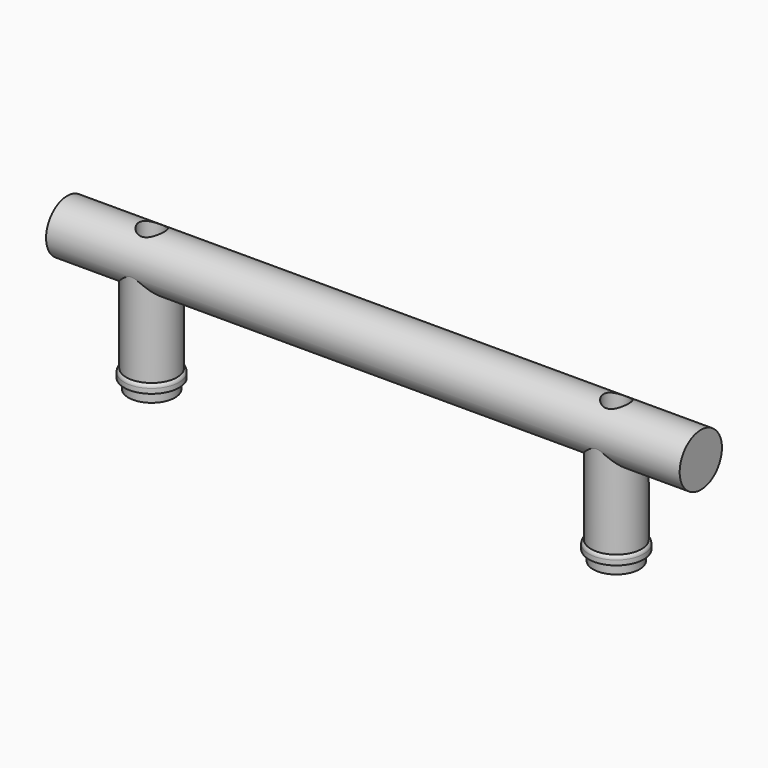
from build123d import *

# Parameters (mm, degrees)
F0_R     = 6
F0_R_2   = 5.5
F0_R_3   = 3
F1_DEPTH = 25
F0_R_4   = 6.5
F2_DEPTH = 2
F0_R_5   = 1.5
F3_DEPTH = 2.4
F4_R     = 6.25
F5_DEPTH = 75
F6_DEPTH = 40


# Not quite as in the source:
# - a fillet or chamfer that OpenCascade refuses, or shapes differently, is made with other operations: its cross-section is extruded or revolved along the edge and cut away or added


with BuildPart() as f1:
    # F0 (on Top) → F1 (new body)
    with BuildSketch(Plane.XY):
        with Locations((-55, 0)):
            Circle(F0_R)
        with Locations((-55, 0)):
            Circle(F0_R_2, mode=Mode.SUBTRACT)
        with Locations((-55, 0)):
            Circle(F0_R_2)
        with Locations((-55, 0)):
            Circle(F0_R_3, mode=Mode.SUBTRACT)
    extrude(amount=F1_DEPTH)

    # F0 (on Top) → F2 (join)
    with BuildSketch(Plane.XY):
        with Locations((-55, 0)):
            Circle(F0_R_4)
        with Locations((-55, 0)):
            Circle(F0_R, mode=Mode.SUBTRACT)
    extrude(amount=F2_DEPTH)

    # F0 (on Top) → F3 (join)
    with BuildSketch(Plane.XY):
        with Locations((-55, 0)):
            Circle(F0_R_2)
        with Locations((-55, 0)):
            Circle(F0_R_3, mode=Mode.SUBTRACT)
        with Locations((-55, 0)):
            Circle(F0_R_3)
        with Locations((-55, 0)):
            Circle(F0_R_5, mode=Mode.SUBTRACT)
    extrude(amount=-F3_DEPTH)

    # F4 (on Right) → F5 (join)
    with BuildSketch(Plane.YZ):
        with Locations((0, 25.1302048564)):
            Circle(F4_R)
    extrude(amount=-F5_DEPTH)

    # F0 (on Top) → F6 (cut)
    with BuildSketch(Plane.XY):
        with Locations((-55, 0)):
            Circle(F0_R_3)
        with Locations((-55, 0)):
            Circle(F0_R_5, mode=Mode.SUBTRACT)
        with Locations((-55, 0)):
            Circle(F0_R_5)
    extrude(amount=F6_DEPTH, mode=Mode.SUBTRACT)

    # F7: fillet of radius 1 on 1 edges, made by hand

    # F7_s1 → F7_t2 (revolve, cut)
    with BuildSketch(Plane.XZ):
        with BuildLine():
            ThreePointArc((-49, 2), (-48.6339745962, 1.6339745962), (-48.5, 1.1339745962))
            Line((-48.5, 1.1339745962), (-48.5, 2))
            Line((-48.5, 2), (-49, 2))
        make_face()
    revolve(axis=Axis((-55, 0, 2), (0, 0, 1)), mode=Mode.SUBTRACT)

    # F8: F1 across plane


with BuildPart() as f1_1:
    add(f1.part)
    add(f1.part.mirror(Plane.YZ))


solid = f1_1.part
